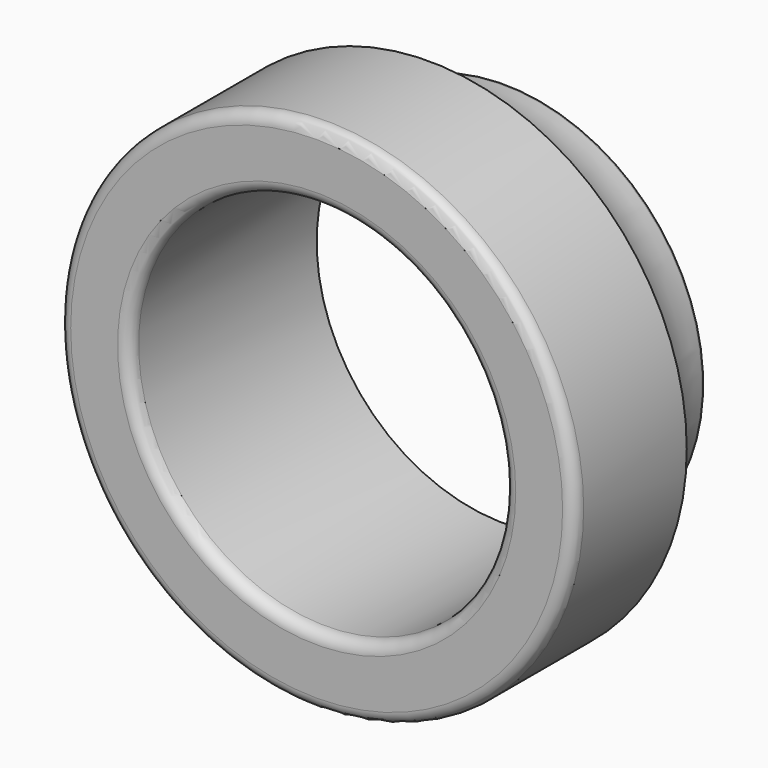
from build123d import *

# Parameters (mm, degrees)
F0_R     = 5.5
F0_R_2   = 4
F4_DEPTH = 5
F5_R     = 0.25
F6_R     = 0.25
F1_R     = 5.5
F1_R_2   = 4.25
F2_DEPTH = 2


# Not quite as in the source:
# - a fillet or chamfer that OpenCascade refuses, or shapes differently, is made with other operations: its cross-section is extruded or revolved along the edge and cut away or added


with BuildPart() as f4:
    # F0 (on Front) → F4 (new body)
    with BuildSketch(Plane.XZ):
        Circle(F0_R)
        Circle(F0_R_2, mode=Mode.SUBTRACT)
    extrude(amount=F4_DEPTH)

    # F5
    f5_edges = [f4.edges().sort_by_distance(p)[0] for p in [
        (-4, -5, 0),
    ]]
    fillet(f5_edges, radius=F5_R)

    # F6
    f6_edges = [f4.edges().sort_by_distance(p)[0] for p in [
        (-5.5, -5, 0),
    ]]
    fillet(f6_edges, radius=F6_R)

    # F1 (on face) → F2 (cut)
    with BuildSketch(Plane(origin=(0, 0, 0), x_dir=(-1, 0, 0), z_dir=(0, 1, 0))):
        Circle(F1_R)
        Circle(F1_R_2, mode=Mode.SUBTRACT)
    extrude(amount=-F2_DEPTH, mode=Mode.SUBTRACT)

    # F3: fillet of radius 2.18 on 1 edges, made by hand

    # F3_s1 → F3_t2 (revolve)
    with BuildSketch(Plane.XY):
        with BuildLine():
            ThreePointArc((-4.25, -0.0283255847), (-4.5888318925, -1.1955873377), (-5.5, -2))
            Line((-5.5, -2), (-5.4814, -2.0394334883))
            ThreePointArc((-5.4814, -2.0394334883), (-4.875, -2.0436), (-4.25, -2.0436))
            Line((-4.25, -2.0436), (-4.2064, -2))
            Line((-4.2064, -2), (-4.2064, -0.0283255847))
            Line((-4.2064, -0.0283255847), (-4.25, -0.0283255847))
        make_face()
    revolve(axis=Axis((0, -2, 0), (0, 1, 0)))


solid = f4.part
